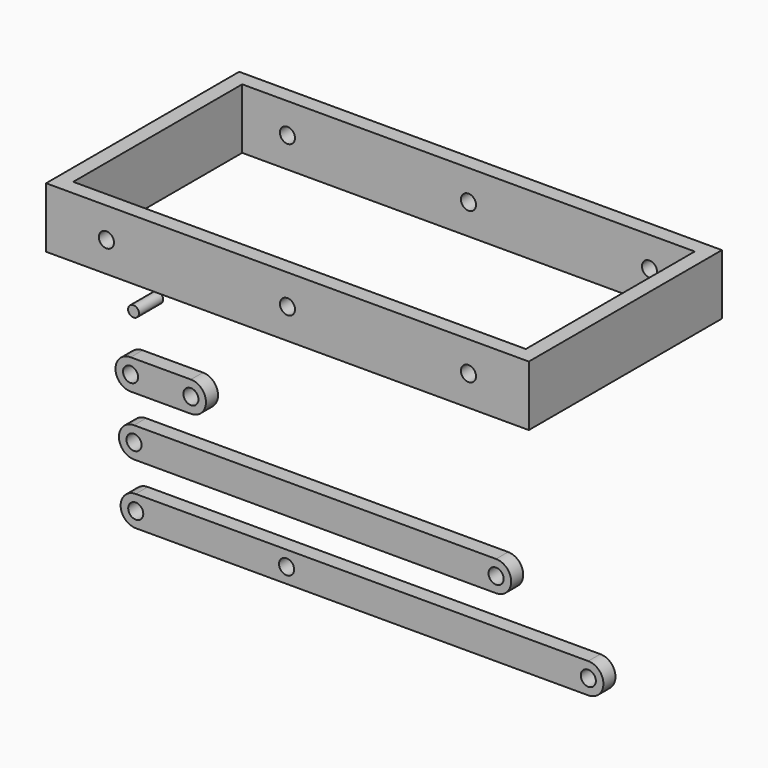
from build123d import *

# Parameters (mm, degrees)
F1_R      = 1.25
F2_DEPTH  = 2.5
F3_R      = 1.25
F4_DEPTH  = 2.5
F5_R      = 1.25
F6_DEPTH  = 2.5
F8_W      = 80
F8_H      = 40
F8_W_2    = 75
F8_H_2    = 35
F9_DEPTH  = 10
F10_R     = 1.25
F11_DEPTH = 40.001
F12_R     = 0.9
F13_DEPTH = 5


with BuildPart() as f2:
    # F1 (on Front) → F2 (new body)
    with BuildSketch(Plane.XZ):
        with BuildLine():
            Line((10, 2.5), (0, 2.5))
            ThreePointArc((0, 2.5), (-2.5, 0), (0, -2.5))
            Line((0, -2.5), (10, -2.5))
            ThreePointArc((10, -2.5), (12.5, 0), (10, 2.5))
        make_face()
        Circle(F1_R, mode=Mode.SUBTRACT)
        with Locations((10, 0)):
            Circle(F1_R, mode=Mode.SUBTRACT)
    extrude(amount=F2_DEPTH)


with BuildPart() as f4:
    # F3 (on Front) → F4 (new body)
    with BuildSketch(Plane.XZ):
        with BuildLine():
            Line((60.5706622079, -7.232673876), (0.5706622079, -7.232673876))
            ThreePointArc((0.5706622079, -7.232673876), (-1.9293377921, -9.732673876), (0.5706622079, -12.232673876))
            Line((0.5706622079, -12.232673876), (60.5706622079, -12.232673876))
            ThreePointArc((60.5706622079, -12.232673876), (63.0706622079, -9.732673876), (60.5706622079, -7.232673876))
        make_face()
        with Locations((0.5706622079, -9.732673876)):
            Circle(F3_R, mode=Mode.SUBTRACT)
        with Locations((60.5706622079, -9.732673876)):
            Circle(F3_R, mode=Mode.SUBTRACT)
    extrude(amount=F4_DEPTH)


with BuildPart() as f6:
    # F5 (on Front) → F6 (new body)
    with BuildSketch(Plane.XZ):
        with BuildLine():
            Line((75.8570737601, -17.1626018733), (0.8570737601, -17.1626018733))
            ThreePointArc((0.8570737601, -17.1626018733), (-1.6429262399, -19.6626018733), (0.8570737601, -22.1626018733))
            Line((0.8570737601, -22.1626018733), (75.8570737601, -22.1626018733))
            ThreePointArc((75.8570737601, -22.1626018733), (78.3570737601, -19.6626018733), (75.8570737601, -17.1626018733))
        make_face()
        with Locations((0.8570737601, -19.6626018733)):
            Circle(F5_R, mode=Mode.SUBTRACT)
        with Locations((25.8570737601, -19.6626018733)):
            Circle(F5_R, mode=Mode.SUBTRACT)
        with Locations((75.8570737601, -19.6626018733)):
            Circle(F5_R, mode=Mode.SUBTRACT)
    extrude(amount=F6_DEPTH)


with BuildPart() as f9:
    # F8 (on offset) → F9 (new body)
    with BuildSketch(Plane.XY.offset(25)):
        with Locations((40, 0)):
            Rectangle(F8_W, F8_H)
        with Locations((40, 0)):
            Rectangle(F8_W_2, F8_H_2, mode=Mode.SUBTRACT)
    extrude(amount=F9_DEPTH)

    # F10 (on face) → F11 (cut, through all)
    with BuildSketch(Plane.XZ.offset(20)):
        with Locations((10, 30)):
            Circle(F10_R)
        with Locations((70, 30)):
            Circle(F10_R)
        with Locations((40, 30)):
            Circle(F10_R)
    extrude(amount=-F11_DEPTH, mode=Mode.SUBTRACT)


with BuildPart() as f13:
    # F12 (on Front) → F13 (new body)
    with BuildSketch(Plane.XZ):
        with Locations((2.488047583, 11.0218990594)):
            Circle(F12_R)
    extrude(amount=F13_DEPTH)


solid = Compound([f2.part, f4.part, f6.part, f9.part, f13.part])
